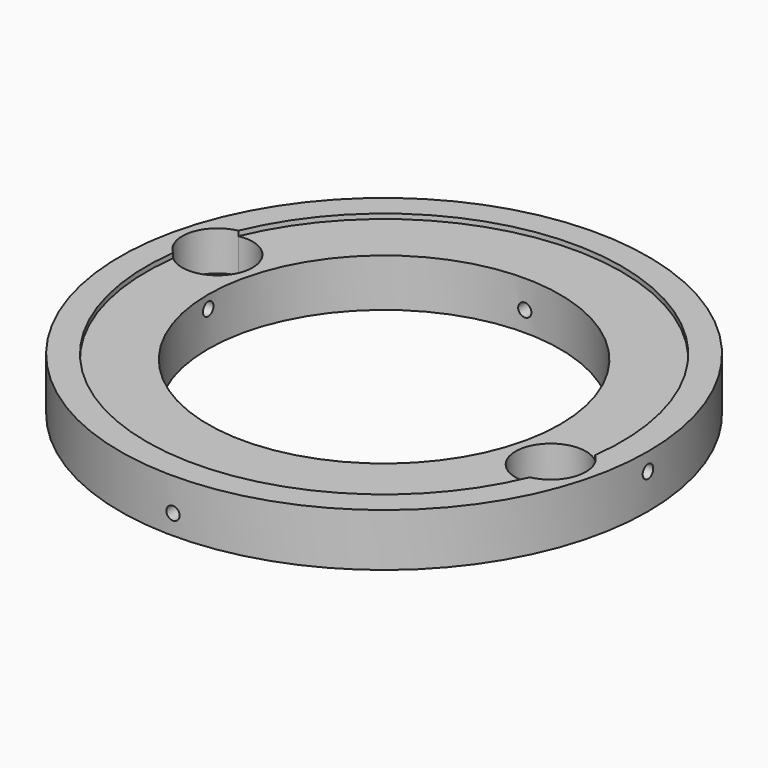
from build123d import *

# Parameters (mm, degrees)
F0_R           = 30
F1_DEPTH       = 6
F2_R           = 27
F3_DEPTH       = 0.55
F4_R           = 0.75
F5_DEPTH       = 30.001
F5_DEPTH_BACK  = 30.001
F6_R           = 20
F7_DEPTH       = 5.4510001
F8_R           = 0.75
F9_DEPTH       = 30.0010001
F9_DEPTH_BACK  = 30.0010001
F11_DEPTH      = 3.95
F11_DEPTH_BACK = 0.5510001
F13_DEPTH      = 4.5
F14_R          = 2.05
F15_DEPTH      = 1.5010001


with BuildPart() as f1:
    # F0 (on Top) → F1 (new body)
    with BuildSketch(Plane.XY):
        Circle(F0_R)
    extrude(amount=F1_DEPTH)

    # F2 (on face) → F3 (cut)
    with BuildSketch(Plane.XY.offset(6)):
        Circle(F2_R)
    extrude(amount=-F3_DEPTH, mode=Mode.SUBTRACT)

    # F4 (on Front) → F5 (cut, two sides)
    with BuildSketch(Plane.XZ) as f5_sk:
        with Locations((0, 2.2661738681)):
            Circle(F4_R)
    extrude(amount=-F5_DEPTH, mode=Mode.SUBTRACT)
    extrude(f5_sk.sketch, amount=F5_DEPTH_BACK, mode=Mode.SUBTRACT)

    # F6 (on face) → F7 (cut, through all)
    with BuildSketch(Plane.XY.offset(5.45)):
        Circle(F6_R)
    extrude(amount=-F7_DEPTH, mode=Mode.SUBTRACT)

    # F8 (on Right) → F9 (cut, two sides)
    with BuildSketch(Plane.YZ) as f9_sk:
        with Locations((0, 4)):
            Circle(F8_R)
    extrude(amount=-F9_DEPTH, mode=Mode.SUBTRACT)
    extrude(f9_sk.sketch, amount=F9_DEPTH_BACK, mode=Mode.SUBTRACT)

    # F10 (on face) → F11 (cut, two sides)
    with BuildSketch(Plane.XY.offset(5.45)) as f11_sk:
        with BuildLine():
            ThreePointArc((-24.9057688902, 10.4260575477), (-28.0026498746, 7.54), (-26.7736042577, 3.4891424523))
            ThreePointArc((-26.7736042577, 3.4891424523), (-26.0714326419, 7.02), (-24.9057688902, 10.4260575477))
        make_face()
        with BuildLine():
            ThreePointArc((24.9057688902, -10.4260575477), (26.0714326419, -7.02), (26.7736042577, -3.4891424523))
            ThreePointArc((26.7736042577, -3.4891424523), (20.2777809437, -5.46), (24.9057688902, -10.4260575477))
        make_face()
    extrude(amount=-F11_DEPTH, mode=Mode.SUBTRACT)
    extrude(f11_sk.sketch, amount=F11_DEPTH_BACK, mode=Mode.SUBTRACT)

    # F12 (on face) → F13 (cut)
    with BuildSketch(Plane.XY.offset(6)):
        with BuildLine():
            ThreePointArc((-26.7736042577, 3.4891424523), (-22.4869694193, 2.8576411905), (-20.1402154091, 6.5))
            ThreePointArc((-20.1402154091, 6.5), (-21.5968135459, 9.587249093), (-24.9057688902, 10.4260575477))
            ThreePointArc((-24.9057688902, 10.4260575477), (-28.0026498746, 7.54), (-26.7736042577, 3.4891424523))
        make_face()
        with BuildLine():
            ThreePointArc((26.7736042577, -3.4891424523), (26.0714326419, -7.02), (24.9057688902, -10.4260575477))
            ThreePointArc((24.9057688902, -10.4260575477), (27.2274645021, -9.0434018632), (28.1402154091, -6.5))
            ThreePointArc((28.1402154091, -6.5), (27.7825742186, -4.8467540102), (26.7736042577, -3.4891424523))
        make_face()
    extrude(amount=-F13_DEPTH, mode=Mode.SUBTRACT)

    # F14 (on face) → F15 (cut, through all)
    with BuildSketch(Plane.XY.offset(1.5)):
        with Locations((-24.1402154091, 6.5)):
            Circle(F14_R)
        with Locations((24.1402154091, -6.5)):
            Circle(F14_R)
    extrude(amount=-F15_DEPTH, mode=Mode.SUBTRACT)


solid = f1.part
